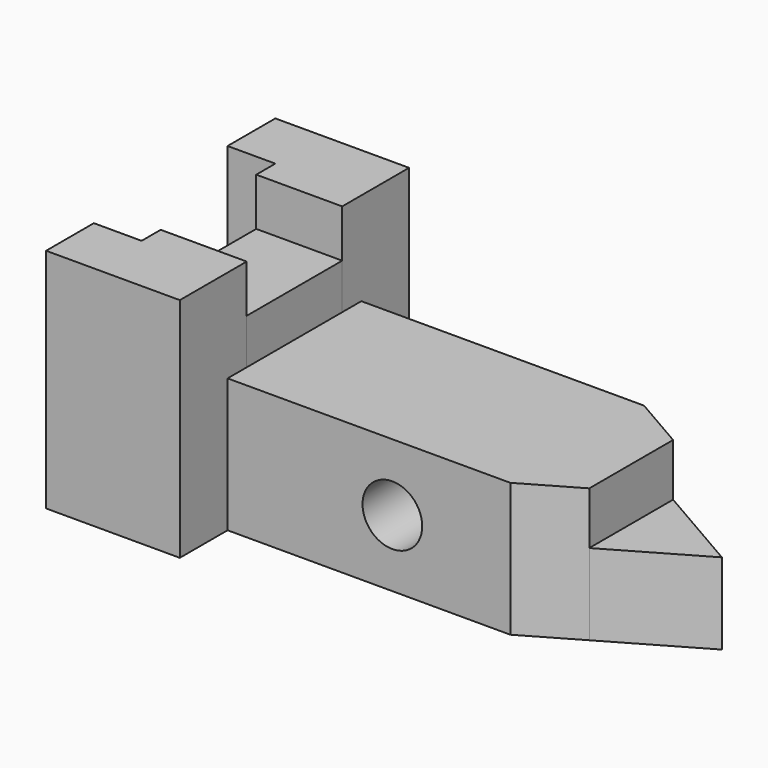
from build123d import *

# Parameters (mm, degrees)
F1_DEPTH = 48.26
F2_DEPTH = 38.1
F3_DEPTH = 28.448
F4_DEPTH = 17.272
F5_R     = 6.35
F6_DEPTH = 71.12


with BuildPart() as f1:
    # F0 (on Top) → F1 (new body)
    with BuildSketch(Plane.XY):
        Polygon((-37.172444715, -25.4), (-55.460444715, -25.4), (-55.460444715, -30.48), (-65.620444715, -30.48), (-65.620444715, -43.18), (-55.460444715, -43.18), (-37.172444715, -43.18), (-37.172444715, -30.48), align=None)
    extrude(amount=F1_DEPTH)


with BuildPart() as f1b:
    # F0 (on Top) → F1, piece 2 (new body)
    with BuildSketch(Plane.XY):
        Polygon((-55.460444715, 17.78), (-65.620444715, 17.78), (-65.620444715, 5.08), (-55.460444715, 5.08), (-55.460444715, 0), (-37.172444715, 0), (-37.172444715, 5.08), (-37.172444715, 17.78), align=None)
    extrude(amount=F1_DEPTH)


with BuildPart() as f2:
    # F0 (on Top) → F2 (new body)
    with BuildSketch(Plane.XY):
        Polygon((-37.172444715, 0), (-55.460444715, 0), (-55.460444715, -25.4), (-37.172444715, -25.4), (-37.172444715, -12.7), align=None)
    extrude(amount=F2_DEPTH)


with BuildPart() as f3:
    # F0 (on Top) → F3 (new body)
    with BuildSketch(Plane.XY):
        Polygon((22.9636919264, 5.08), (-37.172444715, 5.08), (-37.172444715, 0), (-37.172444715, -12.7), (-37.172444715, -25.4), (-37.172444715, -30.48), (22.9636919264, -30.48), (34.455555285, -23.8451695964), (34.455555285, -12.7), (34.455555285, -1.5548304036), align=None)
    extrude(amount=F3_DEPTH)

    # F0 (on Top) → F4 (join)
    with BuildSketch(Plane.XY):
        Polygon((53.759555285, -12.7), (34.455555285, -1.5548304036), (34.455555285, -12.7), (34.455555285, -23.8451695964), align=None)
    extrude(amount=F4_DEPTH)

    # F5 (on face) → F6 (cut)
    with BuildSketch(Plane.XZ.offset(30.48)):
        with Locations((-2.120444715, 14.224)):
            Circle(F5_R)
    extrude(amount=-F6_DEPTH, mode=Mode.SUBTRACT)


solid = Compound([f1.part, f1b.part, f2.part, f3.part])
